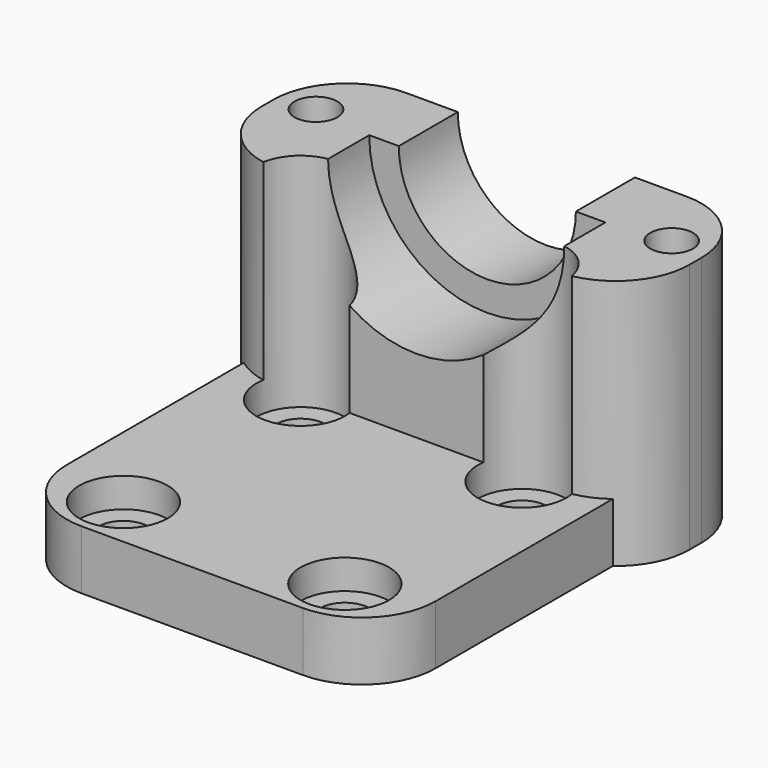
from build123d import *

# Parameters (mm, degrees)
F0_W          = 25
F0_H          = 30
F1_DEPTH      = 4
F2_R          = 1.675
F3_DEPTH      = 25
F4_W          = 25
F4_H          = 11
F5_DEPTH      = 13
F7_DEPTH      = 6
F8_R          = 8
F9_DEPTH      = 6
F2_R_2        = 3
F10_DEPTH     = 2
F11_W         = 11
F11_H         = 17
F12_DEPTH     = 2
F13_R         = 5
F14_W         = 11
F14_H         = 17
F15_DEPTH     = 2
F16_DEPTH     = 2
F17_R         = 1.45
F18_DEPTH     = 25
F19_T1_DEPTH  = 42
F19_T6_DEPTH  = 42
F19_T11_DEPTH = 42
F19_T16_DEPTH = 42
F19_T21_DEPTH = 42
F20_DEPTH     = 25


# Not quite as in the source:
# - a fillet or chamfer that OpenCascade refuses, or shapes differently, is made with other operations: its cross-section is extruded or revolved along the edge and cut away or added


with BuildPart() as f1:
    # F0 (on Top) → F1 (new body)
    with BuildSketch(Plane.XY):
        with Locations((12.5, 15)):
            Rectangle(F0_W, F0_H)
    extrude(amount=F1_DEPTH)

    # F2 (on face) → F3 (cut)
    with BuildSketch(Plane.XY.offset(4)):
        with BuildLine():
            ThreePointArc((3.325, 18.5605346784), (5, 16.8855346784), (6.675, 18.5605346784))
            ThreePointArc((6.675, 18.5605346784), (5, 20.2355346784), (3.325, 18.5605346784))
        make_face()
        with Locations((20, 18.5605346784)):
            Circle(F2_R)
        with Locations((20, 3.5605346784)):
            Circle(F2_R)
        with Locations((5, 3.5605346784)):
            Circle(F2_R)
    extrude(amount=-F3_DEPTH, mode=Mode.SUBTRACT)

    # F4 (on face) → F5 (join)
    with BuildSketch(Plane.XY.offset(4)):
        with Locations((12.5, 24.5)):
            Rectangle(F4_W, F4_H)
    extrude(amount=F5_DEPTH)

    # F6 (on face) → F7 (cut)
    with BuildSketch(Plane(origin=(0, 30, 0), x_dir=(-1, 0, 0), z_dir=(0, 1, 0))):
        with BuildLine():
            ThreePointArc((-18.5, 17), (-12.5, 11), (-6.5, 17))
            Line((-6.5, 17), (-18.5, 17))
        make_face()
    extrude(amount=-F7_DEPTH, mode=Mode.SUBTRACT)

    # F8 (on face) → F9 (cut)
    with BuildSketch(Plane.XZ.offset(-19)):
        with Locations((12.5, 17)):
            Circle(F8_R)
    extrude(amount=-F9_DEPTH, mode=Mode.SUBTRACT)

    # F2 (on face) → F10 (cut)
    with BuildSketch(Plane.XY.offset(4)):
        with BuildLine():
            ThreePointArc((8, 18.5605346784), (5, 21.5605346784), (2, 18.5605346784))
            ThreePointArc((2, 18.5605346784), (5, 15.5605346784), (8, 18.5605346784))
        make_face()
        with BuildLine():
            ThreePointArc((3.325, 18.5605346784), (5, 20.2355346784), (6.675, 18.5605346784))
            ThreePointArc((6.675, 18.5605346784), (5, 16.8855346784), (3.325, 18.5605346784))
        make_face(mode=Mode.SUBTRACT)
        with Locations((20, 18.5605346784)):
            Circle(F2_R_2)
        with Locations((20, 18.5605346784)):
            Circle(F2_R, mode=Mode.SUBTRACT)
        with Locations((20, 3.5605346784)):
            Circle(F2_R_2)
        with Locations((20, 3.5605346784)):
            Circle(F2_R, mode=Mode.SUBTRACT)
        with Locations((5, 3.5605346784)):
            Circle(F2_R_2)
        with Locations((5, 3.5605346784)):
            Circle(F2_R, mode=Mode.SUBTRACT)
    extrude(amount=-F10_DEPTH, mode=Mode.SUBTRACT)

    # F11 (on face) → F12 (join)
    with BuildSketch(Plane(origin=(0, 0, 0), x_dir=(0, -1, 0), z_dir=(-1, 0, 0))):
        with Locations((-24.5, 8.5)):
            Rectangle(F11_W, F11_H)
    extrude(amount=F12_DEPTH)

    # F13
    f13_edges = [f1.edges().sort_by_distance(p)[0] for p in [
        (0, 0, 2),
        (25, 0, 2),
    ]]
    fillet(f13_edges, radius=F13_R)

    # F14 (on face) → F15 (join)
    with BuildSketch(Plane.YZ.offset(25)):
        with Locations((24.5, 8.5)):
            Rectangle(F14_W, F14_H)
    extrude(amount=F15_DEPTH)

    # F14 (on face) → F16 (join)
    with BuildSketch(Plane.YZ.offset(25)):
        with Locations((24.5, 8.5)):
            Rectangle(F14_W, F14_H)
    extrude(amount=F16_DEPTH)

    # F17 (on face) → F18 (cut)
    with BuildSketch(Plane.XY.offset(17)):
        with Locations((0.45, 25.55)):
            Circle(F17_R)
        with Locations((24.55, 25.55)):
            Circle(F17_R)
    extrude(amount=-F18_DEPTH, mode=Mode.SUBTRACT)

    # F19: fillet of radius 5 on 4 edges, made by hand

    # F19_s2 → F19_t1 (cut)
    with BuildSketch(Plane.XY.offset(-12.5)):
        with BuildLine():
            ThreePointArc((-2, 25), (-0.5355339059, 28.5355339059), (3, 30))
            Line((3, 30), (-2, 30))
            Line((-2, 30), (-2, 25))
        make_face()
        with BuildLine():
            ThreePointArc((22, 30), (25.5355339059, 28.5355339059), (27, 25))
            Line((27, 25), (27, 30))
            Line((27, 30), (22, 30))
        make_face()
    extrude(amount=F19_T1_DEPTH, mode=Mode.SUBTRACT)


with BuildPart() as f19_tool4:
    # F19_s5 → F19_t6 (new body)
    with BuildSketch(Plane.XY.offset(-12.5)):
        with BuildLine():
            ThreePointArc((3, 19), (-0.5355339059, 20.4644660941), (-2, 24))
            Line((-2, 24), (-2, 19))
            Line((-2, 19), (3, 19))
        make_face()
    extrude(amount=F19_T6_DEPTH)

    split(bisect_by=Plane.YZ, keep=Keep.BOTTOM)


with BuildPart() as f1_1:
    add(f1.part)

    # F19_t3: cut F19_tool4
    add(f19_tool4.part, mode=Mode.SUBTRACT)


with BuildPart() as f19_tool9:
    # F19_s10 → F19_t11 (new body)
    with BuildSketch(Plane.XY.offset(-12.5)):
        with BuildLine():
            ThreePointArc((3, 19), (-0.5355339059, 20.4644660941), (-2, 24))
            Line((-2, 24), (-2, 19))
            Line((-2, 19), (3, 19))
        make_face()
    extrude(amount=F19_T11_DEPTH)

    split(bisect_by=Plane.XY.offset(4), keep=Keep.TOP)


with BuildPart() as f1_2:
    add(f1_1.part)

    # F19_t8: cut F19_tool9
    add(f19_tool9.part, mode=Mode.SUBTRACT)


with BuildPart() as f19_tool14:
    # F19_s15 → F19_t16 (new body)
    with BuildSketch(Plane.XY.offset(29.5)):
        with BuildLine():
            ThreePointArc((22, 19), (25.5355339059, 20.4644660941), (27, 24))
            Line((27, 24), (27, 19))
            Line((27, 19), (22, 19))
        make_face()
    extrude(amount=-F19_T16_DEPTH)

    split(bisect_by=Plane.XY.offset(4), keep=Keep.TOP)


with BuildPart() as f1_3:
    add(f1_2.part)

    # F19_t13: cut F19_tool14
    add(f19_tool14.part, mode=Mode.SUBTRACT)


with BuildPart() as f19_tool19:
    # F19_s20 → F19_t21 (new body)
    with BuildSketch(Plane.XY.offset(29.5)):
        with BuildLine():
            ThreePointArc((22, 19), (25.5355339059, 20.4644660941), (27, 24))
            Line((27, 24), (27, 19))
            Line((27, 19), (22, 19))
        make_face()
    extrude(amount=-F19_T21_DEPTH)

    split(bisect_by=Plane.YZ.offset(25), keep=Keep.TOP)


with BuildPart() as f1_4:
    add(f1_3.part)

    # F19_t18: cut F19_tool19
    add(f19_tool19.part, mode=Mode.SUBTRACT)

    # F2 (on face) → F20 (cut)
    with BuildSketch(Plane.XY.offset(4)):
        with BuildLine():
            ThreePointArc((8, 18.5605346784), (5, 21.5605346784), (2, 18.5605346784))
            ThreePointArc((2, 18.5605346784), (5, 15.5605346784), (8, 18.5605346784))
        make_face()
        with BuildLine():
            ThreePointArc((3.325, 18.5605346784), (5, 20.2355346784), (6.675, 18.5605346784))
            ThreePointArc((6.675, 18.5605346784), (5, 16.8855346784), (3.325, 18.5605346784))
        make_face(mode=Mode.SUBTRACT)
        with Locations((20, 18.5605346784)):
            Circle(F2_R_2)
        with Locations((20, 18.5605346784)):
            Circle(F2_R, mode=Mode.SUBTRACT)
        with BuildLine():
            ThreePointArc((3.325, 18.5605346784), (5, 16.8855346784), (6.675, 18.5605346784))
            ThreePointArc((6.675, 18.5605346784), (5, 20.2355346784), (3.325, 18.5605346784))
        make_face()
        with Locations((20, 18.5605346784)):
            Circle(F2_R)
    extrude(amount=F20_DEPTH, mode=Mode.SUBTRACT)


solid = f1_4.part
